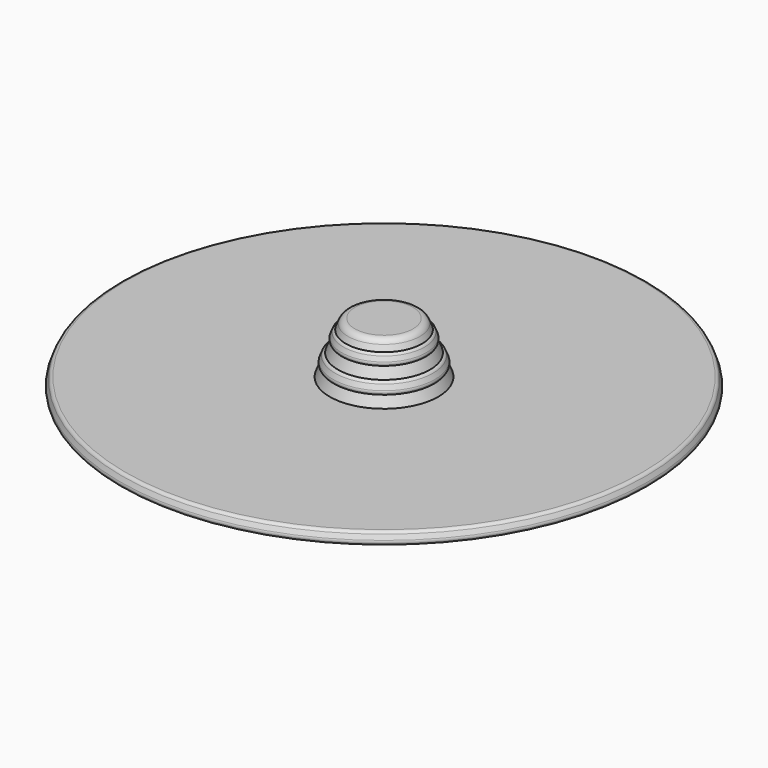
from build123d import *

# Parameters (mm, degrees)
F2_R = 5.08


# Not quite as in the source:
# - a fillet or chamfer that OpenCascade refuses, or shapes differently, is made with other operations: its cross-section is extruded or revolved along the edge and cut away or added


with BuildPart() as f1:
    # F0 (on Front) → F1 (revolve)
    with BuildSketch(Plane.XZ):
        Polygon((23.584696, 48.849477), (0, 48.849477), (0, 47.72635), (22.807644, 47.72635), (60.882603, -44.741469), (184.053146, 5.97578), (181.151834, 13.021828), (37.648683, 13.021828), (34.747372, 20.067876), (36.198225, 20.665286), (33.296913, 27.711333), (31.952542, 27.711333), (29.05123, 34.757381), (30.478069, 34.757381), (27.576757, 41.803429), (26.486008, 41.803429), align=None)
    revolve(axis=Axis((0, 0, 48.287914), (0, 0, 1)))

    # F2
    f2_edges = [f1.edges().sort_by_distance(p)[0] for p in [
        (-23.584696, 0, 48.849477),
    ]]
    fillet(f2_edges, radius=F2_R)

    # F3: fillet of radius 2.54 on 6 edges, made by hand


with BuildPart() as f3_tool1:
    # F3_s2 → F3_t3 (revolve)
    with BuildSketch(Plane.XZ):
        with BuildLine():
            ThreePointArc((26.486008, 41.803429), (27.513225, 41.258876), (28.19019, 40.313661))
            Line((28.19019, 40.313661), (28.237164, 40.333003))
            Line((28.237164, 40.333003), (27.62373, 41.822771))
            Line((27.62373, 41.822771), (27.576757, 41.854229))
            ThreePointArc((27.576757, 41.854229), (27.031382, 41.854229), (26.498898, 41.852566))
            Line((26.498898, 41.852566), (26.486008, 41.803429))
        make_face()
    revolve(axis=Axis((0, 0, 41.803429), (0, 0, 1)))


with BuildPart() as f3_tool4:
    # F3_s5 → F3_t6 (revolve)
    with BuildSketch(Plane.XZ):
        with BuildLine():
            ThreePointArc((29.423108, 37.319429), (29.588085, 35.98747), (29.05123, 34.757381))
            Line((29.05123, 34.757381), (29.090766, 34.725482))
            ThreePointArc((29.090766, 34.725482), (29.764649, 34.706581), (30.478069, 34.706581))
            Line((30.478069, 34.706581), (30.525042, 34.776723))
            Line((30.525042, 34.776723), (29.470082, 37.338771))
            Line((29.470082, 37.338771), (29.423108, 37.319429))
        make_face()
    revolve(axis=Axis((0, 0, 34.757381), (0, 0, 1)))


with BuildPart() as f3_tool7:
    # F3_s8 → F3_t9 (revolve)
    with BuildSketch(Plane.XZ):
        with BuildLine():
            ThreePointArc((31.952542, 27.711333), (33.147657, 27.200414), (33.933561, 26.165188))
            Line((33.933561, 26.165188), (33.980535, 26.18453))
            Line((33.980535, 26.18453), (33.343887, 27.730676))
            Line((33.343887, 27.730676), (33.296913, 27.762133))
            ThreePointArc((33.296913, 27.762133), (32.624728, 27.762133), (31.959895, 27.761598))
            Line((31.959895, 27.761598), (31.952542, 27.711333))
        make_face()
    revolve(axis=Axis((0, 0, 27.711333), (0, 0, 1)))


with BuildPart() as f3_tool10:
    # F3_s11 → F3_t12 (revolve)
    with BuildSketch(Plane.XZ):
        with BuildLine():
            ThreePointArc((35.304572, 22.835588), (35.445929, 21.367185), (34.747372, 20.067876))
            Line((34.747372, 20.067876), (34.783201, 20.031864))
            ThreePointArc((34.783201, 20.031864), (35.49214, 20.319607), (36.217567, 20.618312))
            Line((36.217567, 20.618312), (36.245199, 20.684628))
            Line((36.245199, 20.684628), (35.351545, 22.85493))
            Line((35.351545, 22.85493), (35.304572, 22.835588))
        make_face()
    revolve(axis=Axis((0, 0, 20.665286), (0, 0, 1)))


with BuildPart() as f3_tool13:
    # F3_s14 → F3_t15 (revolve)
    with BuildSketch(Plane.XZ):
        with BuildLine():
            ThreePointArc((179.450814, 13.021828), (180.864171, 12.592283), (181.799497, 11.448932))
            Line((181.799497, 11.448932), (181.84647, 11.468274))
            Line((181.84647, 11.468274), (181.185855, 13.072628))
            Line((181.185855, 13.072628), (179.450814, 13.072628))
            Line((179.450814, 13.072628), (179.450814, 13.021828))
        make_face()
    revolve(axis=Axis((0, 0, 13.021828), (0, 0, 1)))


with BuildPart() as f3_tool16:
    # F3_s17 → F3_t18 (revolve)
    with BuildSketch(Plane.XZ):
        with BuildLine():
            ThreePointArc((183.086042, 8.324463), (183.081975, 6.380435), (181.704463, 5.008676))
            Line((181.704463, 5.008676), (181.723806, 4.961703))
            Line((181.723806, 4.961703), (184.119462, 5.948149))
            Line((184.119462, 5.948149), (183.133016, 8.343805))
            Line((183.133016, 8.343805), (183.086042, 8.324463))
        make_face()
    revolve(axis=Axis((0, 0, 5.97578), (0, 0, 1)))


with BuildPart() as f1_1:
    add(f1.part)

    # F3_t19: cut F3_tool1, F3_tool4, F3_tool7, F3_tool10, F3_tool13, F3_tool16
    add([f3_tool1.part, f3_tool4.part, f3_tool7.part, f3_tool10.part, f3_tool13.part, f3_tool16.part], mode=Mode.SUBTRACT)


solid = f1_1.part
